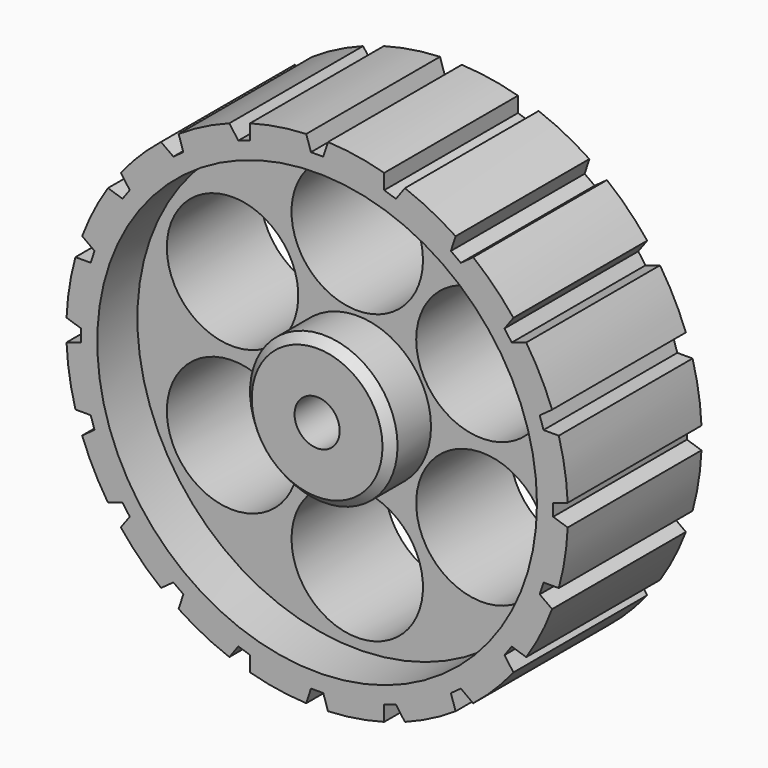
from build123d import *

# Parameters (mm, degrees)
F0_R            = 15
F0_R_2          = 1.35
F1_DEPTH        = 10
F3_R            = 3.9311890732
F4_DEPTH        = 25
F4_COPIES_COUNT = 6
F2_R            = 13.1491583338
F2_R_2          = 4.4111200255
F5_DEPTH        = 3
F6_SIZE         = 0.5
F8_DEPTH        = 10
F9_COUNT        = 20
F10_R           = 3.9505307448
F10_R_2         = 1.35
F11_DEPTH       = 4


# Not quite as in the source:
# - a pattern or mirror of a feature is missing from the dataset's text; its kind, count and spacing are read off the source's solid
# - a feature names something its author has since deleted; it is built from what else it names


with BuildPart() as f1:
    # F0 (on Front) → F1 (new body)
    with BuildSketch(Plane.XZ):
        Circle(F0_R)
        Circle(F0_R_2, mode=Mode.SUBTRACT)
    extrude(amount=F1_DEPTH)

    # F3 (on face) → F4 (cut)
    with BuildSketch(Plane.XZ.offset(10)):
        with Locations((0, 8.6101097986)):
            Circle(F3_R)
    f4 = extrude(amount=-F4_DEPTH, mode=Mode.SUBTRACT)

    # F4_copies: F4 ×6 about axis
    f4_copies_axis = Axis((0, 0, 0), (0, 1, 0))
    for i in range(1, F4_COPIES_COUNT):
        add(f4.rotate(f4_copies_axis, i * 360 / F4_COPIES_COUNT), mode=Mode.SUBTRACT)

    # F2 (on face) → F5 (cut)
    with BuildSketch(Plane.XZ.offset(10)):
        Circle(F2_R)
        Circle(F2_R_2, mode=Mode.SUBTRACT)
    extrude(amount=-F5_DEPTH, mode=Mode.SUBTRACT)

    # F6
    f6_edges = [f1.edges().sort_by_distance(p)[0] for p in [
        (-4.41112, -10, 0),
    ]]
    chamfer(f6_edges, length=F6_SIZE)

    # F7 (on face) → F8 (cut)
    with BuildSketch(Plane.XZ.offset(10)):
        with BuildLine():
            ThreePointArc((0.6504242485, 14.9858916417), (0, 15), (-0.6504242485, 14.9858916417))
            Line((-0.6504242485, 14.9858916417), (-0.3680477384, 14.1178695485))
            Line((-0.3680477384, 14.1178695485), (0, 14.1178695485))
            Line((0, 14.1178695485), (0.3680477384, 14.1178695485))
            Line((0.3680477384, 14.1178695485), (0.6504242485, 14.9858916417))
        make_face()
    f8 = extrude(amount=-F8_DEPTH, mode=Mode.SUBTRACT)

    # F9: F8 ×20 about axis
    f9_axis = Axis((0, 0, 0), (0, 1, 0))
    for i in range(1, F9_COUNT):
        add(f8.rotate(f9_axis, i * 360 / F9_COUNT), mode=Mode.SUBTRACT)

    # F10 (on face) → F11 (join)
    with BuildSketch(Plane(origin=(0, 0, 0), x_dir=(-1, 0, 0), z_dir=(0, 1, 0))):
        Circle(F10_R)
        Circle(F10_R_2, mode=Mode.SUBTRACT)
    extrude(amount=F11_DEPTH)


solid = f1.part
